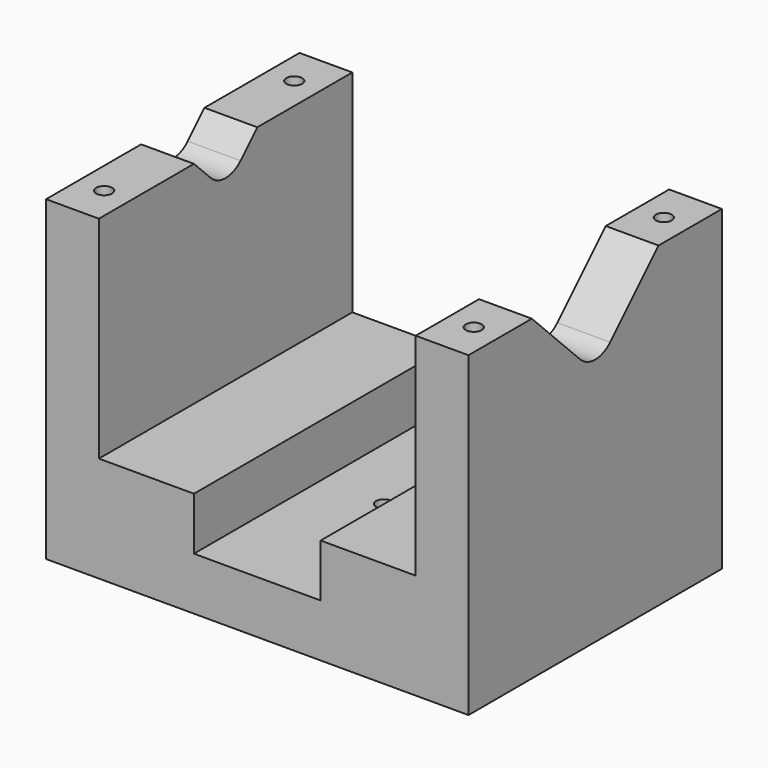
from build123d import *

# Parameters (mm, degrees)
F1_DEPTH  = 60
F3_DEPTH  = 10
F5_DEPTH  = 10
F6_R      = 1.5
F7_R      = 1.5
F8_R      = 1.5
F9_R      = 1.5
F10_DEPTH = 10
F11_R     = 3.5
F12_DEPTH = 4
F13_R     = 1.5
F14_DEPTH = 6


# Not quite as in the source:
# - a feature names something its author has since deleted; it is built from what else it names


with BuildPart() as f1:
    # F0 (on Front) → F1 (new body)
    with BuildSketch(Plane.XZ):
        Polygon((-40, 60), (-40, 0), (40, 0), (40, 60), (30, 60), (30, 20), (12, 20), (12, 10), (-12, 10), (-12, 20), (-30, 20), (-30, 60), align=None)
    extrude(amount=F1_DEPTH)

    # F2 (on face) → F3 (cut, through all)
    with BuildSketch(Plane.YZ.offset(40)):
        with BuildLine():
            ThreePointArc((-33.5355339059, 48.5355339059), (-30, 47.0710678119), (-26.4644660941, 48.5355339059))
            Line((-26.4644660941, 48.5355339059), (-15, 60))
            Line((-15, 60), (-45, 60))
            Line((-45, 60), (-33.5355339059, 48.5355339059))
        make_face()
    extrude(amount=-F3_DEPTH, mode=Mode.SUBTRACT)

    # F4 (on face) → F5 (cut, through all)
    with BuildSketch(Plane(origin=(-40, 0, 0), x_dir=(0, -1, 0), z_dir=(-1, 0, 0))):
        with BuildLine():
            Line((37.5, 60), (22.5, 60))
            Line((22.5, 60), (26.4644660941, 56.0355339059))
            ThreePointArc((26.4644660941, 56.0355339059), (30, 54.5710678119), (33.5355339059, 56.0355339059))
            Line((33.5355339059, 56.0355339059), (37.5, 60))
        make_face()
    extrude(amount=-F5_DEPTH, mode=Mode.SUBTRACT)

    # F6 (on face) + F7 (on face) + F8 (on face) + F9 (on face) → F10 (cut)
    with BuildSketch(Plane.XY.offset(60)):
        with Locations((-35, -7.5)):
            Circle(F6_R)
    with BuildSketch(Plane.XY.offset(60)):
        with Locations((-35, -52.5)):
            Circle(F7_R)
    with BuildSketch(Plane.XY.offset(60)):
        with Locations((35, -7.5)):
            Circle(F8_R)
    with BuildSketch(Plane.XY.offset(60)):
        with Locations((35, -52.5)):
            Circle(F9_R)
    extrude(amount=-F10_DEPTH, mode=Mode.SUBTRACT)

    # F11 (on face) → F12 (cut)
    with BuildSketch(Plane(origin=(0, 0, 0), x_dir=(1, 0, 0), z_dir=(0, 0, -1))):
        with Locations((0, 30)):
            Circle(F11_R)
    extrude(amount=-F12_DEPTH, mode=Mode.SUBTRACT)

    # F13 (on face) → F14 (cut, through all)
    with BuildSketch(Plane(origin=(0, 0, 4), x_dir=(1, 0, 0), z_dir=(0, 0, -1))):
        with Locations((0, 30)):
            Circle(F13_R)
    extrude(amount=-F14_DEPTH, mode=Mode.SUBTRACT)


solid = f1.part
